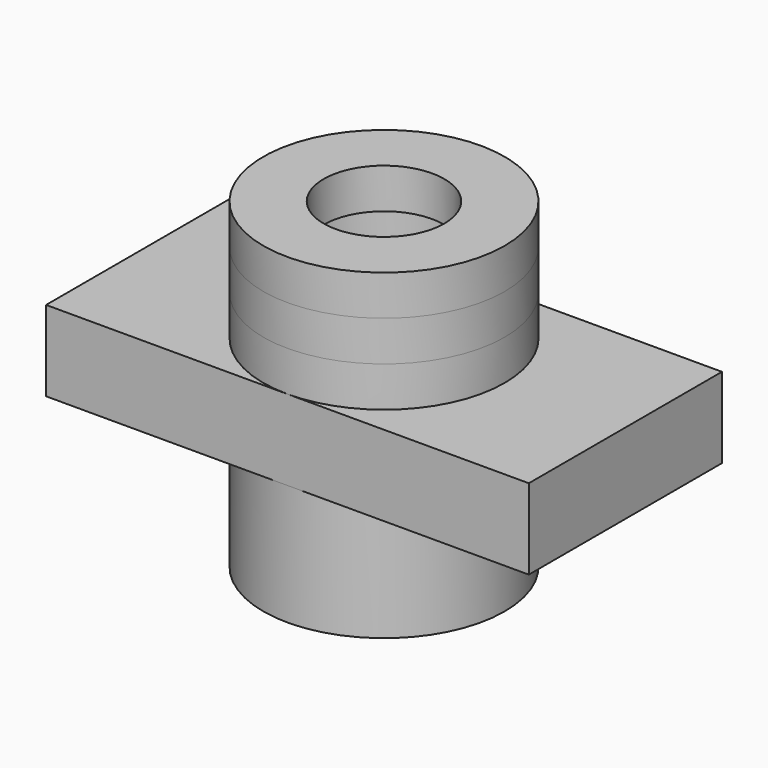
from build123d import *

# Parameters (mm, degrees)
F0_R      = 19.05
F1_DEPTH  = 19.05
F2_W      = 76.2
F2_H      = 38.1
F3_DEPTH  = 12.7
F4_R      = 9.525
F5_DEPTH  = 38.101
F6_R      = 19.05
F7_DEPTH  = 6.35
F8_R      = 12.7
F9_DEPTH  = 6.35
F10_R     = 19.05
F11_DEPTH = 6.35
F12_R     = 9.525
F13_DEPTH = 6.35


# Not quite as in the source:
# - a feature names something its author has since deleted; it is built from what else it names


with BuildPart() as f1:
    # F0 (on Top) → F1 (new body, symmetric)
    with BuildSketch(Plane.XY):
        Circle(F0_R)
    extrude(amount=F1_DEPTH, both=True)

    # F2 (on Top) → F3 (join)
    with BuildSketch(Plane.XY):
        Rectangle(F2_W, F2_H)
    extrude(amount=F3_DEPTH)

    # F4 (on face) → F5 (cut, through all)
    with BuildSketch(Plane.XY.offset(19.05)):
        Circle(F4_R)
    extrude(amount=-F5_DEPTH, mode=Mode.SUBTRACT)

    # F6 (on face) → F7 (join)
    with BuildSketch(Plane.XY.offset(19.05)):
        Circle(F6_R)
    extrude(amount=F7_DEPTH)

    # F8 (on face) → F9 (cut)
    with BuildSketch(Plane.XY.offset(25.4)):
        Circle(F8_R)
    extrude(amount=-F9_DEPTH, mode=Mode.SUBTRACT)

    # F10 (on face) → F11 (join)
    with BuildSketch(Plane.XY.offset(25.4)):
        Circle(F10_R)
    extrude(amount=F11_DEPTH)

    # F12 (on face) → F13 (cut)
    with BuildSketch(Plane.XY.offset(31.75)):
        Circle(F12_R)
    extrude(amount=-F13_DEPTH, mode=Mode.SUBTRACT)


solid = f1.part
